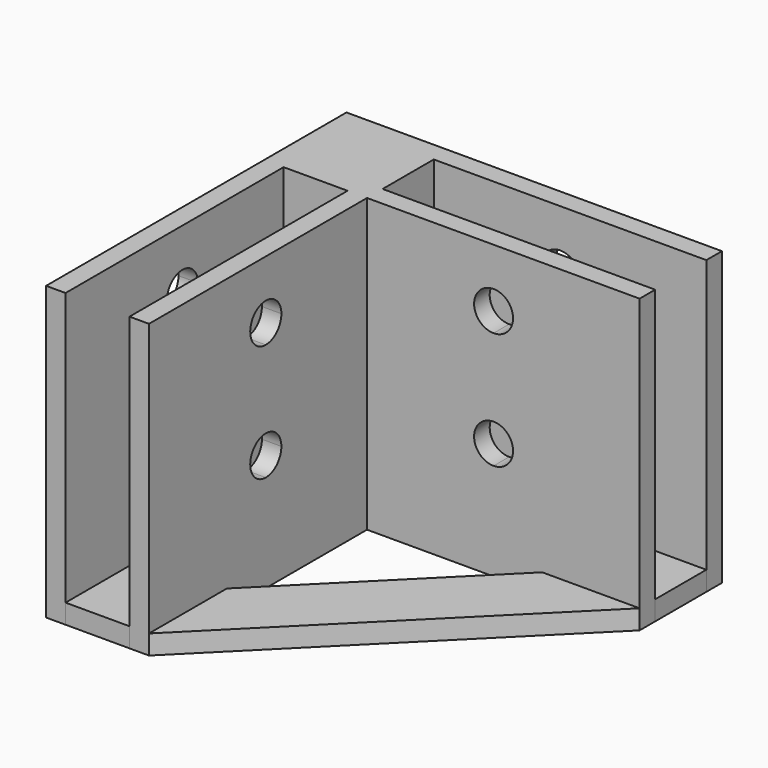
from build123d import *

# Parameters (mm, degrees)
F0_W     = 2
F0_H     = 2
F0_W_2   = 28
F0_H_2   = 28
F1_DEPTH = 30
F0_H_3   = 6.57
F2_DEPTH = 2
F0_W_3   = 6.57
F4_DEPTH = 2
F6_DEPTH = 20
F8_DEPTH = 25


# Not quite as in the source:
# - a feature names something its author has since deleted; it is built from what else it names


with BuildPart() as f1:
    # F0 (on Top) → F1 (new body)
    with BuildSketch(Plane.XY):
        Polygon((-6.57, -2), (-6.57, 6.57), (-8.57, 6.57), (-8.57, -30), (-6.57, -30), align=None)
        with Locations((-7.57, 7.57)):
            Rectangle(F0_W, F0_H)
        Polygon((2, 6.57), (30, 6.57), (30, 8.57), (-6.57, 8.57), (-6.57, 6.57), align=None)
        with Locations((16, -1)):
            Rectangle(F0_W_2, F0_H)
        with Locations((1, -16)):
            Rectangle(F0_W, F0_H_2)
        with Locations((1, -1)):
            Rectangle(F0_W, F0_H)
        Polygon((0, 0), (2, 0), (2, 6.57), (-6.57, 6.57), (-6.57, -2), (0, -2), align=None)
    extrude(amount=F1_DEPTH)


with BuildPart() as f2:
    # F0 (on Top) → F2 (new body)
    with BuildSketch(Plane.XY):
        with Locations((16, 3.285)):
            Rectangle(F0_W_2, F0_H_3)
    extrude(amount=F2_DEPTH)


with BuildPart() as f2b:
    # F0 (on Top) → F2, piece 2 (new body)
    with BuildSketch(Plane.XY):
        with Locations((-3.285, -16)):
            Rectangle(F0_W_3, F0_H_2)
    extrude(amount=F2_DEPTH)


with BuildPart() as f4:
    # F3 (on face) → F4 (new body)
    with BuildSketch(Plane(origin=(0, 0, 0), x_dir=(1, 0, 0), z_dir=(0, 0, -1))):
        Polygon((20, 2), (30, 2), (2, 30), (2, 20), align=None)
    extrude(amount=-F4_DEPTH)


with BuildPart() as f6:
    # F5 (on face) → F6 (new body)
    with BuildSketch(Plane.YZ.offset(2)):
        with BuildLine():
            ThreePointArc((-13, 24), (-16.4142135624, 25.4142135624), (-15, 22))
            ThreePointArc((-15, 22), (-13.5857864376, 22.5857864376), (-13, 24))
        make_face()
    extrude(amount=-F6_DEPTH)


with BuildPart() as f6b:
    # F5 (on face) → F6, piece 2 (new body)
    with BuildSketch(Plane.YZ.offset(2)):
        with BuildLine():
            Line((-15, 12), (-15, 10))
            ThreePointArc((-15, 10), (-13.5857864376, 10.5857864376), (-13, 12))
            ThreePointArc((-13, 12), (-13.5857864376, 13.4142135624), (-15, 14))
            Line((-15, 14), (-15, 12))
        make_face()
        with BuildLine():
            ThreePointArc((-15, 14), (-17, 12), (-15, 10))
            Line((-15, 10), (-15, 12))
            Line((-15, 12), (-15, 14))
        make_face()
    extrude(amount=-F6_DEPTH)


with BuildPart() as f8:
    # F7 (on face) → F8 (new body)
    with BuildSketch(Plane.XZ.offset(2)):
        with BuildLine():
            ThreePointArc((17, 24), (13.5857864376, 25.4142135624), (15, 22))
            ThreePointArc((15, 22), (16.4142135624, 22.5857864376), (17, 24))
        make_face()
    extrude(amount=-F8_DEPTH)


with BuildPart() as f8b:
    # F7 (on face) → F8, piece 2 (new body)
    with BuildSketch(Plane.XZ.offset(2)):
        with BuildLine():
            ThreePointArc((15, 14), (13, 12), (15, 10))
            Line((15, 10), (15, 12))
            Line((15, 12), (15, 14))
        make_face()
        with BuildLine():
            Line((15, 12), (15, 10))
            ThreePointArc((15, 10), (16.4142135624, 10.5857864376), (17, 12))
            ThreePointArc((17, 12), (16.4142135624, 13.4142135624), (15, 14))
            Line((15, 14), (15, 12))
        make_face()
    extrude(amount=-F8_DEPTH)


with BuildPart() as f1_1:
    add(f1.part)

    # F9: cut F8, F6, F6b, F8b
    add(f8.part, mode=Mode.SUBTRACT)
    add(f6.part, mode=Mode.SUBTRACT)
    add(f6b.part, mode=Mode.SUBTRACT)
    add(f8b.part, mode=Mode.SUBTRACT)


solid = Compound([f2.part, f2b.part, f4.part, f1_1.part])
